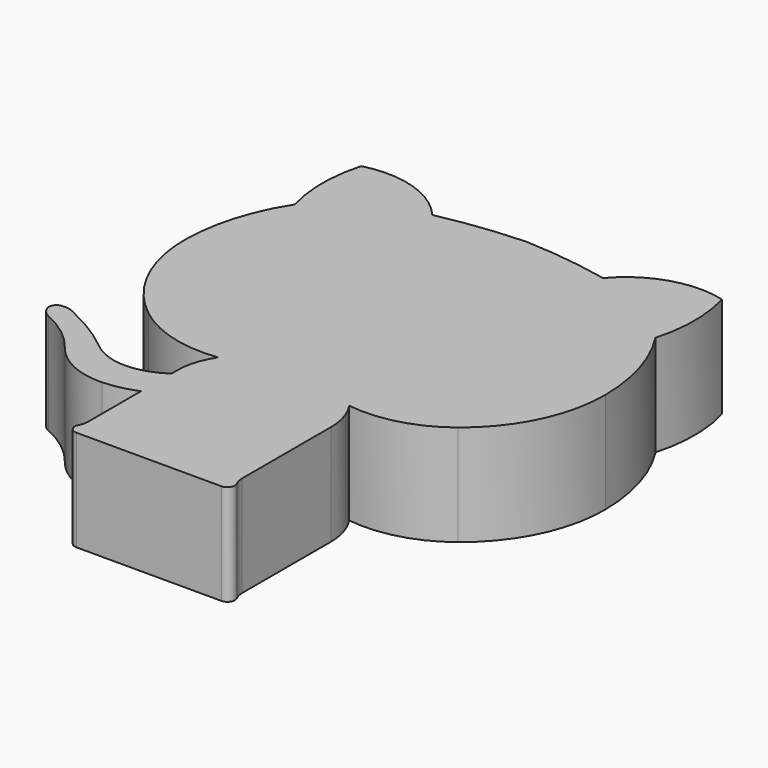
from build123d import *

# Parameters (mm, degrees)
F1_DEPTH    = 4
F3_DEPTH    = 4
F4_T1_DEPTH = 8.9373301178
F4_T3_DEPTH = 5.4979166118


# Not quite as in the source:
# - a fillet or chamfer that OpenCascade refuses, or shapes differently, is made with other operations: its cross-section is extruded or revolved along the edge and cut away or added


with BuildPart() as f1:
    # F0 (on Top) → F1 (new body)
    with BuildSketch(Plane.XY):
        with BuildLine():
            Line((5.4043182717, 11.9166336954), (9.2633608729, 11.9166336954))
            Line((9.2633608729, 11.9166336954), (13.1224034741, 11.9166336954))
            ThreePointArc((13.1224034741, 11.9166336954), (12.5478266836, 12.1546311946), (12.3098291843, 12.7292079851))
            Line((12.3098291843, 12.7292079851), (12.3098291843, 17.1262745588))
            ThreePointArc((12.3098291843, 17.1262745588), (12.1943632439, 17.8955690891), (11.8581410497, 18.5970682651))
            ThreePointArc((11.8581410497, 18.5970682651), (13.7265197912, 18.7234015951), (15.3986439109, 19.5664912462))
            ThreePointArc((15.3986439109, 19.5664912462), (17.0218223076, 21.5886397467), (17.5903830677, 24.1185668856))
            ThreePointArc((17.5903830677, 24.1185668856), (17.2823984437, 26.1835910199), (16.4102166891, 28.0805565417))
            ThreePointArc((16.4102166891, 28.0805565417), (16.638828313, 29.724361375), (16.4102166891, 31.3681662083))
            ThreePointArc((16.4102166891, 31.3681662083), (14.3575671426, 31.3236587754), (12.6471198819, 30.1879998296))
            ThreePointArc((12.6471198819, 30.1879998296), (10.9641887914, 30.4698973914), (9.2633608729, 30.6074026007))
            ThreePointArc((9.2633608729, 30.6074026007), (7.5625329544, 30.4698973914), (5.8796018638, 30.1879998296))
            ThreePointArc((5.8796018638, 30.1879998296), (4.1691546032, 31.3236587754), (2.1165050566, 31.3681662083))
            ThreePointArc((2.1165050566, 31.3681662083), (1.8878934327, 29.724361375), (2.1165050566, 28.0805565417))
            ThreePointArc((2.1165050566, 28.0805565417), (1.244323302, 26.1835910199), (0.936338678, 24.1185668856))
            ThreePointArc((0.936338678, 24.1185668856), (1.5048994381, 21.5886397467), (3.1280778348, 19.5664912462))
            ThreePointArc((3.1280778348, 19.5664912462), (4.8002019546, 18.7234015951), (6.668580696, 18.5970682651))
            ThreePointArc((6.668580696, 18.5970682651), (6.3323585018, 17.8955690891), (6.2168925614, 17.1262745588))
            Line((6.2168925614, 17.1262745588), (6.2168925614, 12.7292079851))
            ThreePointArc((6.2168925614, 12.7292079851), (5.9788950622, 12.1546311946), (5.4043182717, 11.9166336954))
        make_face()
    extrude(amount=F1_DEPTH)

    # F2 (on Top) → F3 (join, through all)
    with BuildSketch(Plane.XY):
        with BuildLine():
            ThreePointArc((6.2168925614, 16.8439224371), (5.6798309181, 16.5586654348), (5.0929421559, 16.3993909955))
            ThreePointArc((5.0929421559, 16.3993909955), (4.1545493311, 16.4529754412), (3.3199274912, 16.8852470815))
            ThreePointArc((3.3199274912, 16.8852470815), (2.3265556072, 17.5975106191), (1.2477898737, 18.1722901762))
            ThreePointArc((1.2477898737, 18.1722901762), (0.8448717213, 18.2802980548), (0.441953569, 18.1722901762))
            ThreePointArc((0.441953569, 18.1722901762), (0.5289468082, 17.7574058892), (0.8448717213, 17.4747608034))
            ThreePointArc((0.8448717213, 17.4747608034), (1.7862867621, 16.9138981945), (2.5603426512, 16.1382264689))
            ThreePointArc((2.5603426512, 16.1382264689), (3.5961993789, 15.3105799436), (4.8955686661, 15.0466909773))
            ThreePointArc((4.8955686661, 15.0466909773), (5.5689958467, 15.1314623043), (6.2168925614, 15.3337497048))
            Line((6.2168925614, 15.3337497048), (6.2168925614, 16.8439224371))
        make_face()
    extrude(amount=F3_DEPTH)

    # F4: fillet of radius 0.3 on 3 edges, made by hand

    # F4_s2 → F4_t1 (cut)
    with BuildSketch(Plane.XY.offset(-2.4686650589)):
        with BuildLine():
            ThreePointArc((12.1349374505, 11.9166336954), (12.3913198946, 12.0608516606), (12.4012026427, 12.3548467462))
            ThreePointArc((12.4012026427, 12.3548467462), (12.7004552198, 12.0347753771), (13.1224034741, 11.9166336954))
            Line((13.1224034741, 11.9166336954), (12.1349374505, 11.9166336954))
        make_face()
        with BuildLine():
            ThreePointArc((6.1255191031, 12.3548467462), (6.1354018511, 12.0608516606), (6.3917842952, 11.9166336954))
            Line((6.3917842952, 11.9166336954), (5.4043182717, 11.9166336954))
            ThreePointArc((5.4043182717, 11.9166336954), (5.8262665259, 12.0347753771), (6.1255191031, 12.3548467462))
        make_face()
    extrude(amount=F4_T1_DEPTH, mode=Mode.SUBTRACT)

    # F4_s4 → F4_t3 (cut)
    with BuildSketch(Plane.XY.offset(-0.7489583059)):
        with BuildLine():
            ThreePointArc((0.7077089455, 18.2685344716), (0.5003837706, 18.1253146023), (0.4753670818, 17.8745760445))
            ThreePointArc((0.4753670818, 17.8745760445), (0.4420534576, 18.0215692627), (0.441953569, 18.1722901762))
            ThreePointArc((0.441953569, 18.1722901762), (0.5705770014, 18.2321594237), (0.7077089455, 18.2685344716))
        make_face()
    extrude(amount=F4_T3_DEPTH, mode=Mode.SUBTRACT)


solid = f1.part
